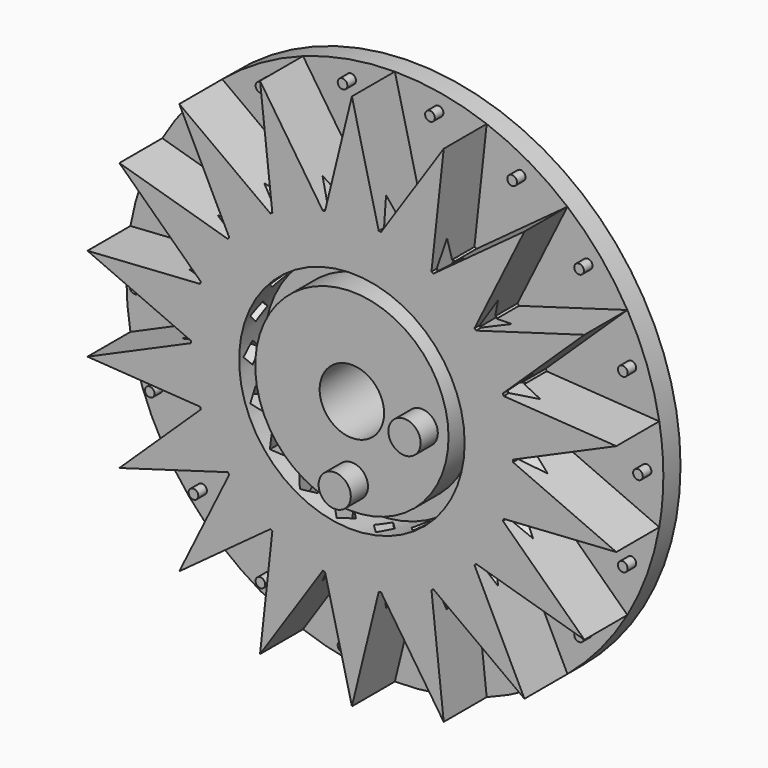
from build123d import *

# Parameters (mm, degrees)
F0_R      = 25
F1_DEPTH  = 2
F2_R      = 15
F3_DEPTH  = 5
F4_R      = 3
F5_DEPTH  = 5
F7_DEPTH  = 5
F8_ANGLE  = -20
F9_ANGLE  = -20
F10_ANGLE = -20
F11_ANGLE = -20
F14_R     = 0.45
F15_DEPTH = 1
F16_ANGLE = 20
F17_ANGLE = 20
F18_ANGLE = 20
F19_ANGLE = 20
F20_ANGLE = 20
F23_R     = 10.5
F23_R_2   = 9
F24_DEPTH = 3
F28_DEPTH = 5
F30_ANGLE = 10
F31_ANGLE = 20
F32_ANGLE = 20
F33_ANGLE = 20
F34_ANGLE = 20
F38_R     = 1.5
F39_DEPTH = 2


with BuildPart() as f1:
    # F0 (on Front) → F1 (new body)
    with BuildSketch(Plane.XZ):
        Circle(F0_R)
    extrude(amount=-F1_DEPTH)

    # F2 (on Front) → F3 (join)
    with BuildSketch(Plane.XZ):
        Circle(F2_R)
    extrude(amount=F3_DEPTH)

    # F4 (on Front) → F5 (cut, symmetric)
    with BuildSketch(Plane.XZ):
        Circle(F4_R)
    extrude(amount=F5_DEPTH, both=True, mode=Mode.SUBTRACT)

    # F6 (on Front) → F7 (join)
    with BuildSketch(Plane.XZ):
        with BuildLine():
            ThreePointArc((-2.5, 14.7901994577), (0, 15), (2.5, 14.7901994577))
            Line((2.5, 14.7901994577), (0, 25))
            Line((0, 25), (-2.5, 14.7901994577))
        make_face()
    extrude(amount=F7_DEPTH)


with BuildPart() as f8_1:
    # F8: copy of F1
    add(f1.part.rotate(Axis((0, 0, 0), (0, -1, 0)), F8_ANGLE))


with BuildPart() as f9_1:
    # F9: copy of F8_1
    add(f8_1.part.rotate(Axis((0, 0, 0), (0, -1, 0)), F9_ANGLE))


with BuildPart() as f10_1:
    # F10: copy of F9_1
    add(f9_1.part.rotate(Axis((0, 0, 0), (0, -1, 0)), F10_ANGLE))


with BuildPart() as f11_1:
    # F11: copy of F10_1
    add(f10_1.part.rotate(Axis((0, 0, 0), (0, -1, 0)), F11_ANGLE))


with BuildPart() as f12_1:
    # F12: instance of F1
    add(f1.part.mirror(Plane.YZ))


with BuildPart() as f12_2:
    # F12: instance of F8_1
    add(f8_1.part.mirror(Plane.YZ))


with BuildPart() as f12_3:
    # F12: instance of F9_1
    add(f9_1.part.mirror(Plane.YZ))


with BuildPart() as f12_4:
    # F12: instance of F10_1
    add(f10_1.part.mirror(Plane.YZ))


with BuildPart() as f12_5:
    # F12: instance of F11_1
    add(f11_1.part.mirror(Plane.YZ))


with BuildPart() as f1_1:
    add(f1.part)

    add(f8_1.part)  # F13 merges F8_1

    add(f9_1.part)  # F13 merges F9_1

    add(f10_1.part)  # F13 merges F10_1

    add(f11_1.part)  # F13 merges F11_1

    add(f12_1.part)  # F13 merges F12_1

    add(f12_2.part)  # F13 merges F12_2

    add(f12_3.part)  # F13 merges F12_3

    add(f12_4.part)  # F13 merges F12_4

    add(f12_5.part)  # F13 merges F12_5
    # F13: F12_5, F12_4, F12_3, F12_2, F12_1, F8_1, F9_1, F10_1, F11_1 across plane
    add(f12_5.part.mirror(Plane.XY))
    add(f12_4.part.mirror(Plane.XY))
    add(f12_3.part.mirror(Plane.XY))
    add(f12_2.part.mirror(Plane.XY))
    add(f12_1.part.mirror(Plane.XY))
    add(f8_1.part.mirror(Plane.XY))
    add(f9_1.part.mirror(Plane.XY))
    add(f10_1.part.mirror(Plane.XY))
    add(f11_1.part.mirror(Plane.XY))

    # F14 (on face) → F15 (join)
    with BuildSketch(Plane.XZ):
        with Locations((4.0694992911, 23.0792773443)):
            Circle(F14_R)
    extrude(amount=F15_DEPTH)


with BuildPart() as f16_1:
    # F16: copy of F1
    add(f1_1.part.rotate(Axis((0, 0, 0), (0, -1, 0)), F16_ANGLE))


with BuildPart() as f17_1:
    # F17: copy of F16_1
    add(f16_1.part.rotate(Axis((0, 0, 0), (0, -1, 0)), F17_ANGLE))


with BuildPart() as f18_1:
    # F18: copy of F17_1
    add(f17_1.part.rotate(Axis((0, 0, 0), (0, -1, 0)), F18_ANGLE))


with BuildPart() as f19_1:
    # F19: copy of F18_1
    add(f18_1.part.rotate(Axis((0, 0, 0), (0, -1, 0)), F19_ANGLE))


with BuildPart() as f20_1:
    # F20: copy of F19_1
    add(f19_1.part.rotate(Axis((0, 0, 0), (0, -1, 0)), F20_ANGLE))


with BuildPart() as f21_1:
    # F21: instance of F19_1
    add(f19_1.part.mirror(Plane.XY))


with BuildPart() as f21_2:
    # F21: instance of F18_1
    add(f18_1.part.mirror(Plane.XY))


with BuildPart() as f21_3:
    # F21: instance of F17_1
    add(f17_1.part.mirror(Plane.XY))


with BuildPart() as f21_4:
    # F21: instance of F16_1
    add(f16_1.part.mirror(Plane.XY))


with BuildPart() as f1_2:
    add(f1_1.part)

    add(f16_1.part)  # F22 merges F16_1

    add(f17_1.part)  # F22 merges F17_1

    add(f18_1.part)  # F22 merges F18_1

    add(f19_1.part)  # F22 merges F19_1

    add(f20_1.part)  # F22 merges F20_1

    add(f21_1.part)  # F22 merges F21_1

    add(f21_2.part)  # F22 merges F21_2

    add(f21_3.part)  # F22 merges F21_3

    add(f21_4.part)  # F22 merges F21_4
    # F22: F21_4, F21_3, F21_2, F21_1, F20_1, F19_1, F18_1, F17_1 across plane
    add(f21_4.part.mirror(Plane.YZ))
    add(f21_3.part.mirror(Plane.YZ))
    add(f21_2.part.mirror(Plane.YZ))
    add(f21_1.part.mirror(Plane.YZ))
    add(f20_1.part.mirror(Plane.YZ))
    add(f19_1.part.mirror(Plane.YZ))
    add(f18_1.part.mirror(Plane.YZ))
    add(f17_1.part.mirror(Plane.YZ))


with BuildPart() as f24:
    # F23 (on Front) → F24 (new body)
    with BuildSketch(Plane.XZ):
        Circle(F23_R)
        Circle(F23_R_2, mode=Mode.SUBTRACT)
    extrude(amount=F24_DEPTH)


with BuildPart() as f24_1:
    # F25: moved
    add(f24.part.moved(Location((0, -2.07, 0))))


with BuildPart() as f1_3:
    add(f1_2.part)

    # F26: cut F24
    add(f24_1.part, mode=Mode.SUBTRACT)

    # F36: F28, F31_1, F32_1, F35_3, F35_2, F35_1, F33_1, F34_1, F35_4 across plane


with BuildPart() as f28:
    # F27 (on Top) → F28 (new body, symmetric)
    with BuildSketch(Plane.XY):
        Polygon((0, -3.6), (1, -2.6), (0, -1.6), (-1, -2.6), align=None)
    extrude(amount=F28_DEPTH, both=True)


with BuildPart() as f28_1:
    # F29: moved
    add(f28.part.moved(Location((0, -0.89, 15))))


with BuildPart() as f28_2:
    # F30: moved
    add(f28_1.part.rotate(Axis((0, 0, 0), (0, -1, 0)), F30_ANGLE))


with BuildPart() as f31_1:
    # F31: copy of F28
    add(f28_2.part.rotate(Axis((0, 0, 0), (0, -1, 0)), F31_ANGLE))


with BuildPart() as f32_1:
    # F32: copy of F31_1
    add(f31_1.part.rotate(Axis((0, 0, 0), (0, -1, 0)), F32_ANGLE))


with BuildPart() as f33_1:
    # F33: copy of F32_1
    add(f32_1.part.rotate(Axis((0, 0, 0), (0, -1, 0)), F33_ANGLE))


with BuildPart() as f34_1:
    # F34: copy of F33_1
    add(f33_1.part.rotate(Axis((0, 0, 0), (0, -1, 0)), F34_ANGLE))


with BuildPart() as f35_1:
    # F35: instance of F28
    add(f28_2.part.mirror(Plane.XY))


with BuildPart() as f35_2:
    # F35: instance of F31_1
    add(f31_1.part.mirror(Plane.XY))


with BuildPart() as f35_3:
    # F35: instance of F32_1
    add(f32_1.part.mirror(Plane.XY))


with BuildPart() as f35_4:
    # F35: instance of F33_1
    add(f33_1.part.mirror(Plane.XY))


with BuildPart() as f1_4:
    add(f1_3.part)
    add(f28_2.part.mirror(Plane.YZ), mode=Mode.SUBTRACT)
    add(f31_1.part.mirror(Plane.YZ), mode=Mode.SUBTRACT)
    add(f32_1.part.mirror(Plane.YZ), mode=Mode.SUBTRACT)
    add(f35_3.part.mirror(Plane.YZ), mode=Mode.SUBTRACT)
    add(f35_2.part.mirror(Plane.YZ), mode=Mode.SUBTRACT)
    add(f35_1.part.mirror(Plane.YZ), mode=Mode.SUBTRACT)
    add(f33_1.part.mirror(Plane.YZ), mode=Mode.SUBTRACT)
    add(f34_1.part.mirror(Plane.YZ), mode=Mode.SUBTRACT)
    add(f35_4.part.mirror(Plane.YZ), mode=Mode.SUBTRACT)

    # F37: cut F28, F31_1, F32_1, F33_1, F35_4, F35_3, F35_2, F35_1, F34_1
    add(f28_2.part, mode=Mode.SUBTRACT)
    add(f31_1.part, mode=Mode.SUBTRACT)
    add(f32_1.part, mode=Mode.SUBTRACT)
    add(f33_1.part, mode=Mode.SUBTRACT)
    add(f35_4.part, mode=Mode.SUBTRACT)
    add(f35_3.part, mode=Mode.SUBTRACT)
    add(f35_2.part, mode=Mode.SUBTRACT)
    add(f35_1.part, mode=Mode.SUBTRACT)
    add(f34_1.part, mode=Mode.SUBTRACT)

    # F38 (on face) → F39 (join)
    with BuildSketch(Plane.XZ.offset(5)):
        with Locations((6.5, 0)):
            Circle(F38_R)
        with Locations((0, -6.5)):
            Circle(F38_R)
    extrude(amount=F39_DEPTH)


solid = f1_4.part
